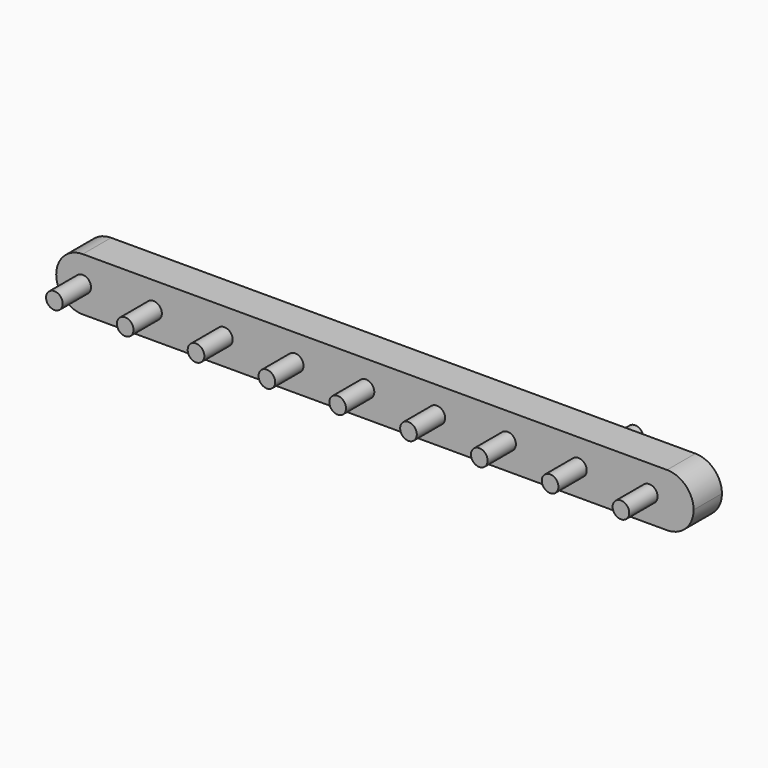
from build123d import *

# Parameters (mm, degrees)
F0_W     = 228.6
F0_H     = 19.05
F0_R     = 2.9845
F1_DEPTH = 12.7
F2_DEPTH = 25.4
F3_R     = 2.9845
F4_DEPTH = 12.7
F5_R     = 9.52499


# Not quite as in the source:
# - a fillet or chamfer is up to 0.001 mm smaller than in the source, because OpenCascade refuses the exact size
# - a feature names something its author has since deleted; it is built from what else it names


with BuildPart() as f1:
    # F0 (on Front) → F1 (new body)
    with BuildSketch(Plane.XZ):
        with Locations((3.2032227146, 0)):
            Rectangle(F0_W, F0_H)
        with Locations((-101.6, 0)):
            Circle(F0_R, mode=Mode.SUBTRACT)
        with Locations((-76.2, 0)):
            Circle(F0_R, mode=Mode.SUBTRACT)
        with Locations((-50.8, 0)):
            Circle(F0_R, mode=Mode.SUBTRACT)
        with Locations((-25.4, 0)):
            Circle(F0_R, mode=Mode.SUBTRACT)
        Circle(F0_R, mode=Mode.SUBTRACT)
        with Locations((25.4, 0)):
            Circle(F0_R, mode=Mode.SUBTRACT)
        with Locations((50.8, 0)):
            Circle(F0_R, mode=Mode.SUBTRACT)
        with Locations((76.2, 0)):
            Circle(F0_R, mode=Mode.SUBTRACT)
        with Locations((101.6, 0)):
            Circle(F0_R, mode=Mode.SUBTRACT)
    extrude(amount=F1_DEPTH)

    # F0 (on Front) → F2 (join)
    with BuildSketch(Plane.XZ):
        Circle(F0_R)
        with Locations((-101.6, 0)):
            Circle(F0_R)
        with Locations((-76.2, 0)):
            Circle(F0_R)
        with Locations((-50.8, 0)):
            Circle(F0_R)
        with Locations((-25.4, 0)):
            Circle(F0_R)
        with Locations((25.4, 0)):
            Circle(F0_R)
        with Locations((50.8, 0)):
            Circle(F0_R)
        with Locations((76.2, 0)):
            Circle(F0_R)
        with Locations((101.6, 0)):
            Circle(F0_R)
    extrude(amount=F2_DEPTH)

    # F3 (on face) → F4 (join)
    with BuildSketch(Plane(origin=(0, 0, 0), x_dir=(-1, 0, 0), z_dir=(0, 1, 0))):
        with Locations((-76.2, 0)):
            Circle(F3_R)
    extrude(amount=F4_DEPTH)

    # F5 (radius 9.525 in the source; OpenCascade refuses exactly that, so slightly less here)
    f5_edges = [f1.edges().sort_by_distance(p)[0] for p in [
        (117.503223, -6.35, 9.525),
        (117.503223, -6.35, -9.525),
        (-111.096777, -6.35, 9.525),
        (-111.096777, -6.35, -9.525),
    ]]
    fillet(f5_edges, radius=F5_R)


solid = f1.part
